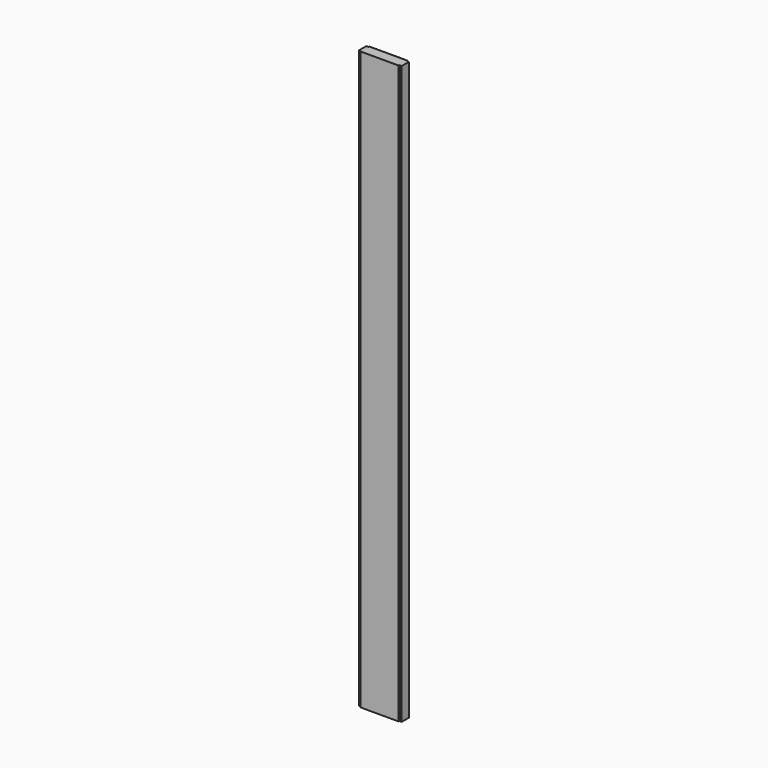
from build123d import *

# Parameters (mm, degrees)
F0_W     = 45
F0_H     = 9.5
F1_DEPTH = 609.6
F2_W     = 40
F2_H     = 609.6
F3_DEPTH = 1


with BuildPart() as f1:
    # F0 (on Top) → F1 (new body)
    with BuildSketch(Plane.XY):
        Rectangle(F0_W, F0_H)
    extrude(amount=F1_DEPTH)


with BuildPart() as f3:
    # F2 (on face) → F3 (new body)
    with BuildSketch(Plane.XZ.offset(4.75)):
        with Locations((0, 304.8)):
            Rectangle(F2_W, F2_H)
    extrude(amount=F3_DEPTH)


with BuildPart() as f4_1:
    # F4: instance of F3
    add(f3.part.mirror(Plane.XZ))


solid = Compound([f1.part, f3.part, f4_1.part])
